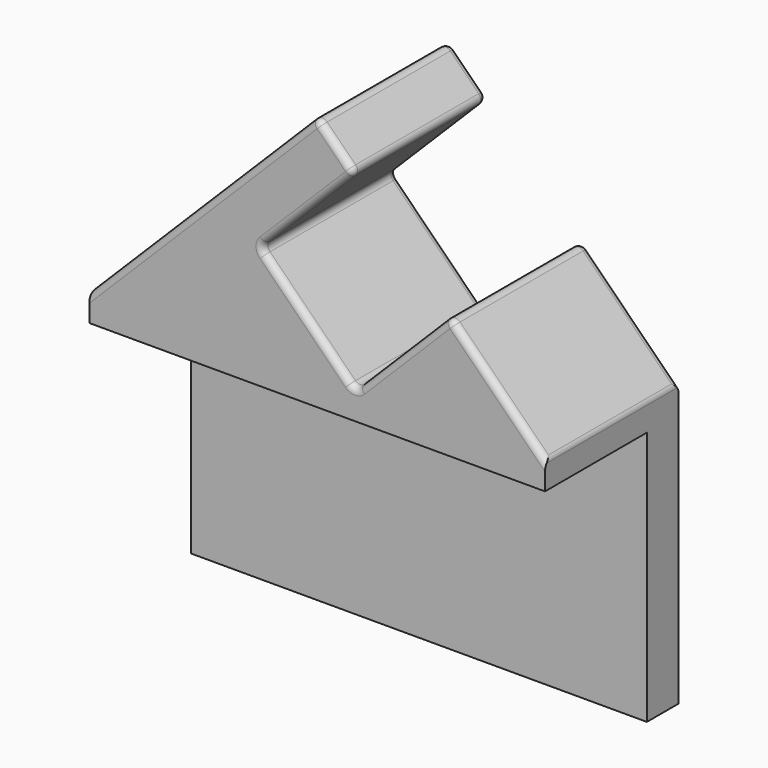
from build123d import *

# Parameters (mm, degrees)
F1_DEPTH    = 25
F2_W        = 19.05
F2_H        = 38.1
F3_DEPTH    = 68.1660937064
F4_F1_R     = 1
F4_F2_R     = 1
F5_R        = 5
F5_R_2      = 1.5875
F6_DEPTH    = 37.6693332908
F7_DEPTH    = 10
F8_S5_R     = 5
F8_T6_DEPTH = 10
F9_R        = 0.5


# Not quite as in the source:
# - a fillet or chamfer that OpenCascade refuses, or shapes differently, is made with other operations: its cross-section is extruded or revolved along the edge and cut away or added


with BuildPart() as f1:
    # F0 (on Front) → F1 (new body)
    with BuildSketch(Plane.XZ):
        Polygon((-34.0825468532, 76.1825468532), (-68.1650937064, 42.1), (-68.1650937064, 0), (0, 0), (0, 42.1), (-14.2128463018, 56.3128463018), (-28.4256926037, 42.1), (-42.6385389055, 56.3128463018), (-28.4256926037, 70.5256926037), align=None)
    extrude(amount=F1_DEPTH)

    # F2 (on face) → F3 (cut, through all)
    with BuildSketch(Plane.YZ):
        with Locations((-15.475, 19.05)):
            Rectangle(F2_W, F2_H)
    extrude(amount=-F3_DEPTH, mode=Mode.SUBTRACT)

    # F4: fillet of radius 1 on 17 edges, made by hand

    # F4_f1
    f4_f1_edges = [f1.edges().sort_by_distance(p)[0] for p in [
        (-42.6385389055, -12.5, 56.3128463018),
        (-28.4256926037, -12.5, 42.1),
    ]]
    fillet(f4_f1_edges, radius=F4_F1_R)

    # F4_f2
    f4_f2_edges = [f1.edges().sort_by_distance(p)[0] for p in [
        (-28.4256926037, -12.5, 70.5256926037),
        (-35.178562364, 0, 63.7728228434),
        (-35.178562364, -25, 63.7728228434),
        (-14.2128463018, -12.5, 56.3128463018),
        (-20.9657160622, 0, 49.5599765415),
        (-20.9657160622, -25, 49.5599765415),
        (-34.0825468532, -12.5, 76.1825468532),
        (-68.1650937064, -12.5, 42.1),
        (-51.1238202798, 0, 59.1412734266),
        (-51.1238202798, -25, 59.1412734266),
        (0, -12.5, 42.1),
        (-7.1064231509, 0, 49.2064231509),
        (-7.1064231509, -25, 49.2064231509),
        (-31.2541197284, 0, 73.3541197284),
        (-31.2541197284, -25, 73.3541197284),
        (-28.4256926037, -25, 42.5142135624),
        (-28.4256926037, 0, 42.5142135624),
        (-42.2243253432, -25, 56.3128463018),
        (-42.2243253432, 0, 56.3128463018),
    ]]
    fillet(f4_f2_edges, radius=F4_F2_R)

    # F5 (on face) → F6 (cut, through all)
    with BuildSketch(Plane(origin=(0, 0, 38.1), x_dir=(1, 0, 0), z_dir=(0, 0, -1))):
        with Locations((-56.1650937064, 15.475)):
            Circle(F5_R)
        with Locations((-56.1650937064, 15.475)):
            Circle(F5_R_2, mode=Mode.SUBTRACT)
        with Locations((-56.1650937064, 15.475)):
            Circle(F5_R_2)
    extrude(amount=-F6_DEPTH, mode=Mode.SUBTRACT)

    # F5 (on face) → F7 (join)
    with BuildSketch(Plane(origin=(0, 0, 38.1), x_dir=(1, 0, 0), z_dir=(0, 0, -1))):
        with Locations((-56.1650937064, 15.475)):
            Circle(F5_R)
        with Locations((-56.1650937064, 15.475)):
            Circle(F5_R_2, mode=Mode.SUBTRACT)
    extrude(amount=-F7_DEPTH)

    # F8: chamfer of 4 on 1 edges, made by hand


with BuildPart() as f8_tool2:
    # F8_s3 → F8_t4 (revolve)
    with BuildSketch(Plane.XZ.offset(15.475)):
        Polygon((-54.5775937064, 44.1), (-50.5775937064, 48.1), (-54.5775937064, 48.1), align=None)
    revolve(axis=Axis((-56.1650937064, -15.475, 48.1), (0, 0, -1)))

    # F8_s5 → F8_t6 (intersect, symmetric)
    with BuildSketch(Plane.XY.offset(46.1)):
        with Locations((-56.1650937064, -15.475)):
            Circle(F8_S5_R)
    extrude(amount=F8_T6_DEPTH, both=True, mode=Mode.INTERSECT)


with BuildPart() as f1_1:
    add(f1.part)

    # F8_t1: cut F8_tool2
    add(f8_tool2.part, mode=Mode.SUBTRACT)

    # F9
    f9_edges = [f1_1.edges().sort_by_distance(p)[0] for p in [
        (-61.165093, -15.47181, 49.100001),
        (-51.165094, -15.475, 53.30625),
        (-61.165094, -15.475, 47.5125),
        (-57.752594, -15.475, 44.1),
    ]]
    fillet(f9_edges, radius=F9_R)


solid = f1_1.part
